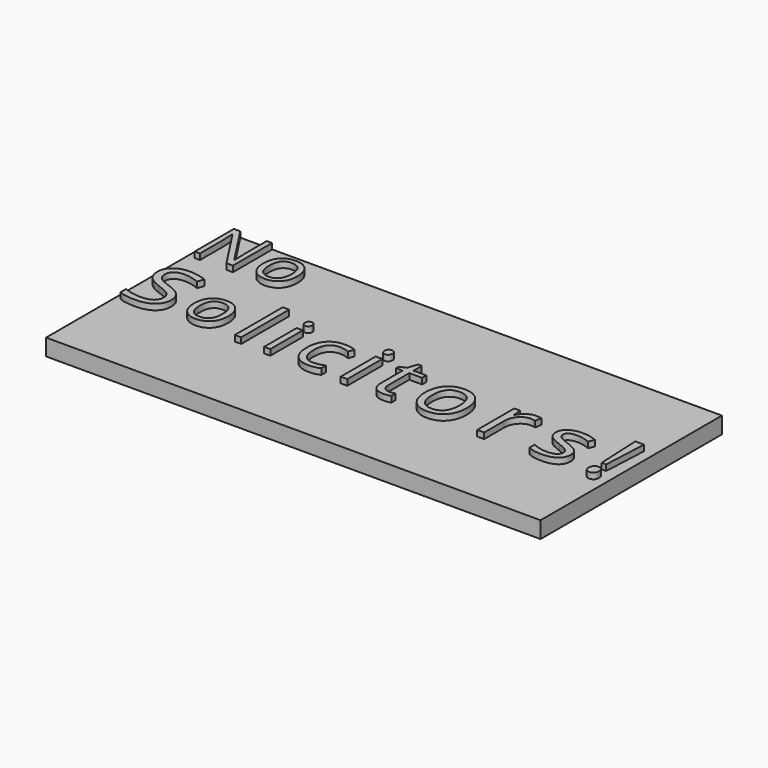
from build123d import *

# Parameters (mm, degrees)
F0_W            = 128.5406574607
F0_H            = 58.9363295585
F1_DEPTH        = 4.318
F2_TEXT_SIZE    = 17.806059236
F2_TEXT_SIZE_2  = 18.2514629909
F2_TEXT_SIZE_3  = 22.679244738
F2_TEXT_SIZE_4  = 20.4851132973
F2_TEXT_SIZE_5  = 19.7844483261
F2_TEXT_SIZE_6  = 21.1507754607
F2_TEXT_SIZE_7  = 21.232162059
F2_TEXT_SIZE_8  = 21.5984673964
F2_TEXT_SIZE_9  = 22.2172788603
F2_TEXT_SIZE_10 = 22.5527755295
F2_TEXT_SIZE_11 = 22.5220606404
F2_TEXT_SIZE_12 = 22.4331781889
F3_DEPTH        = 1.524


# Not quite as in the source:
# - Text() gives the source's letters only with a copy of the font that has no kerning and outlines rounded to 1/6400 em; it was checked with that copy


with BuildPart() as f1:
    # F0 (on Top) → F1 (new body)
    with BuildSketch(Plane.XY):
        with Locations((1.9237361848, 3.0604926869)):
            Rectangle(F0_W, F0_H)
    extrude(amount=-F1_DEPTH)

    # F2 (on face) → F3 (join)
    with BuildSketch(Plane.XY):
        with Locations((-62.3465925455, 19.7082948163)):
            Text('N', F2_TEXT_SIZE, font='Open Sans', text_align=(TextAlign.LEFT, TextAlign.BOTTOM))
        with Locations((-47.4875669555, 19.3876041128)):
            Text('o', F2_TEXT_SIZE_2, font='Open Sans', text_align=(TextAlign.LEFT, TextAlign.BOTTOM))
        with Locations((-62.3465925455, -4.2085159667)):
            Text('S', F2_TEXT_SIZE_3, font='Open Sans', text_align=(TextAlign.LEFT, TextAlign.BOTTOM))
        with Locations((-47.4875669555, -3.1107955274)):
            Text('o', F2_TEXT_SIZE_2, font='Open Sans', text_align=(TextAlign.LEFT, TextAlign.BOTTOM))
        with Locations((-33.0864768475, -3.8538402878)):
            Text('l', F2_TEXT_SIZE_4, font='Open Sans', text_align=(TextAlign.LEFT, TextAlign.BOTTOM))
        with Locations((-25.1176865773, -4.2145449687)):
            Text('i', F2_TEXT_SIZE_5, font='Open Sans', text_align=(TextAlign.LEFT, TextAlign.BOTTOM))
        with Locations((-17.6484531257, -4.6987272799)):
            Text('c', F2_TEXT_SIZE_6, font='Open Sans', text_align=(TextAlign.LEFT, TextAlign.BOTTOM))
        with Locations((-4.9091523979, -4.7573256306)):
            Text('i', F2_TEXT_SIZE_7, font='Open Sans', text_align=(TextAlign.LEFT, TextAlign.BOTTOM))
        with Locations((3.0678561889, -5.0210654736)):
            Text('t', F2_TEXT_SIZE_8, font='Open Sans', text_align=(TextAlign.LEFT, TextAlign.BOTTOM))
        with Locations((13.362351805, -5.4666097276)):
            Text('o', F2_TEXT_SIZE_9, font='Open Sans', text_align=(TextAlign.LEFT, TextAlign.BOTTOM))
        with Locations((31.2247723341, -5.7081673294)):
            Text('r', F2_TEXT_SIZE_10, font='Open Sans', text_align=(TextAlign.LEFT, TextAlign.BOTTOM))
        with Locations((45.1334118843, -5.6860526092)):
            Text('s', F2_TEXT_SIZE_11, font='Open Sans', text_align=(TextAlign.LEFT, TextAlign.BOTTOM))
        with Locations((59.5186799765, -5.6220572442)):
            Text('!', F2_TEXT_SIZE_12, font='Open Sans', text_align=(TextAlign.LEFT, TextAlign.BOTTOM))
    extrude(amount=F3_DEPTH)


solid = f1.part
